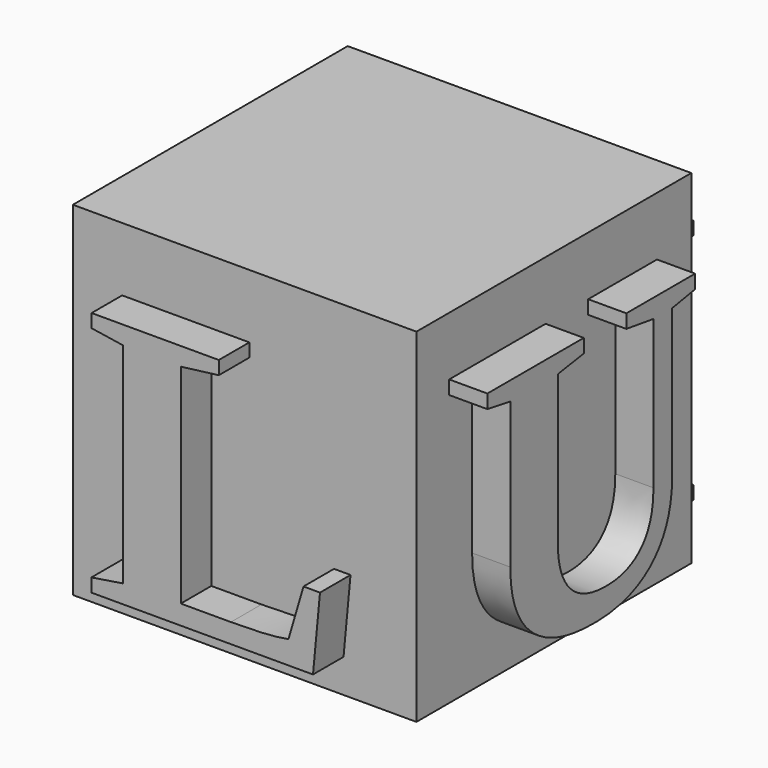
from build123d import *

# Parameters (mm, degrees)
F0_W         = 22.86
F0_H         = 22.86
F1_DEPTH     = 22.86
F2_TEXT_SIZE = 25.0183881157
F3_DEPTH     = 2.54
F4_TEXT_SIZE = 25.6958753905
F5_DEPTH     = 2.54
F6_TEXT_SIZE = 25.0162906013
F7_DEPTH     = 2.54
F8_TEXT_SIZE = 25.5429496368
F9_DEPTH     = 2.54


# Not quite as in the source:
# - Text() gives the source's letters only with a copy of the font that has no kerning and outlines rounded to 1/6400 em; it was checked with that copy


with BuildPart() as f1:
    # F0 (on Front) → F1 (new body)
    with BuildSketch(Plane.XZ):
        Rectangle(F0_W, F0_H)
    extrude(amount=F1_DEPTH)

    # F2 (on face) → F3 (join)
    with BuildSketch(Plane.XZ.offset(22.86)):
        with Locations((-8.5924726736, -9.1969722251)):
            Text('L', F2_TEXT_SIZE, font='Tinos', font_style=FontStyle.BOLD, text_align=(TextAlign.LEFT, TextAlign.BOTTOM))
    extrude(amount=F3_DEPTH)

    # F4 (on face) → F5 (join)
    with BuildSketch(Plane.YZ.offset(11.43)):
        with Locations((-20.775437355, -9.3023693189)):
            Text('U', F4_TEXT_SIZE, font='Tinos', font_style=FontStyle.BOLD, text_align=(TextAlign.LEFT, TextAlign.BOTTOM))
    extrude(amount=F5_DEPTH)

    # F6 (on face) → F7 (join)
    with BuildSketch(Plane(origin=(0, 0, 0), x_dir=(-1, 0, 0), z_dir=(0, 1, 0))):
        with Locations((-9.9537633359, -9.3850590783)):
            Text('K', F6_TEXT_SIZE, font='Tinos', font_style=FontStyle.BOLD, text_align=(TextAlign.LEFT, TextAlign.BOTTOM))
    extrude(amount=F7_DEPTH)

    # F8 (on face) → F9 (join)
    with BuildSketch(Plane(origin=(-11.43, 0, 0), x_dir=(0, -1, 0), z_dir=(-1, 0, 0))):
        with Locations((2.1803674754, -9.1954618692)):
            Text('E', F8_TEXT_SIZE, font='Tinos', font_style=FontStyle.BOLD, text_align=(TextAlign.LEFT, TextAlign.BOTTOM))
    extrude(amount=F9_DEPTH)


solid = f1.part
